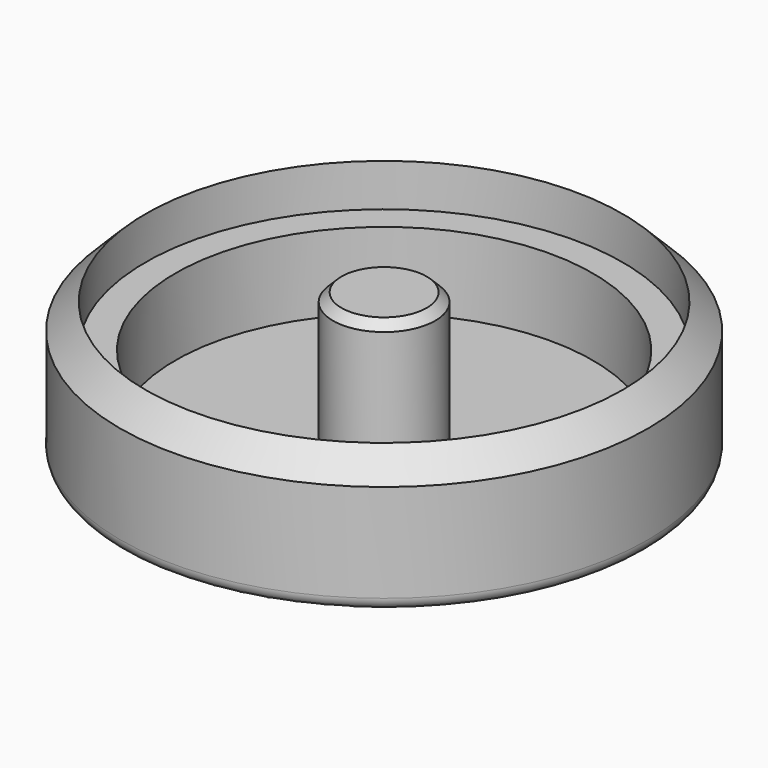
from build123d import *

# Parameters (mm, degrees)
F0_R     = 12.4
F0_R_2   = 9.8
F1_DEPTH = 3.6
F2_R     = 12.4
F2_R_2   = 9.8
F3_DEPTH = 0.8
F4_R     = 12.4
F4_R_2   = 11.2
F5_DEPTH = 2
F6_R     = 0.6
F7_R     = 2.4
F8_DEPTH = 6
F9_SIZE  = 0.4


# Not quite as in the source:
# - a fillet or chamfer that OpenCascade refuses, or shapes differently, is made with other operations: its cross-section is extruded or revolved along the edge and cut away or added


with BuildPart() as f1:
    # F0 (on Top) → F1 (new body)
    with BuildSketch(Plane.XY):
        Circle(F0_R)
        Circle(F0_R_2, mode=Mode.SUBTRACT)
    extrude(amount=F1_DEPTH)

    # F2 (on face) → F3 (join)
    with BuildSketch(Plane(origin=(0, 0, 0), x_dir=(1, 0, 0), z_dir=(0, 0, -1))):
        Circle(F2_R)
        Circle(F2_R_2, mode=Mode.SUBTRACT)
        Circle(F2_R_2)
    extrude(amount=F3_DEPTH)

    # F4 (on face) → F5 (join)
    with BuildSketch(Plane.XY.offset(3.6)):
        Circle(F4_R)
        Circle(F4_R_2, mode=Mode.SUBTRACT)
    extrude(amount=F5_DEPTH)

    # F6
    f6_edges = [f1.edges().sort_by_distance(p)[0] for p in [
        (-12.4, 0, -0.8),
    ]]
    fillet(f6_edges, radius=F6_R)

    # F7 (on face) → F8 (join)
    with BuildSketch(Plane.XY):
        Circle(F7_R)
    extrude(amount=F8_DEPTH)

    # F9
    f9_edges = [f1.edges().sort_by_distance(p)[0] for p in [
        (-2.4, 0, 6),
    ]]
    chamfer(f9_edges, length=F9_SIZE)

    # F10: chamfer of 1.2 on 1 edges, made by hand

    # F10_s1 → F10_t2 (revolve, cut)
    with BuildSketch(Plane.XZ):
        Polygon((11.2, 5.6), (12.4, 4.4), (12.4, 5.6), align=None)
    revolve(axis=Axis((0, 0, 5.6), (0, 0, 1)), mode=Mode.SUBTRACT)


solid = f1.part
